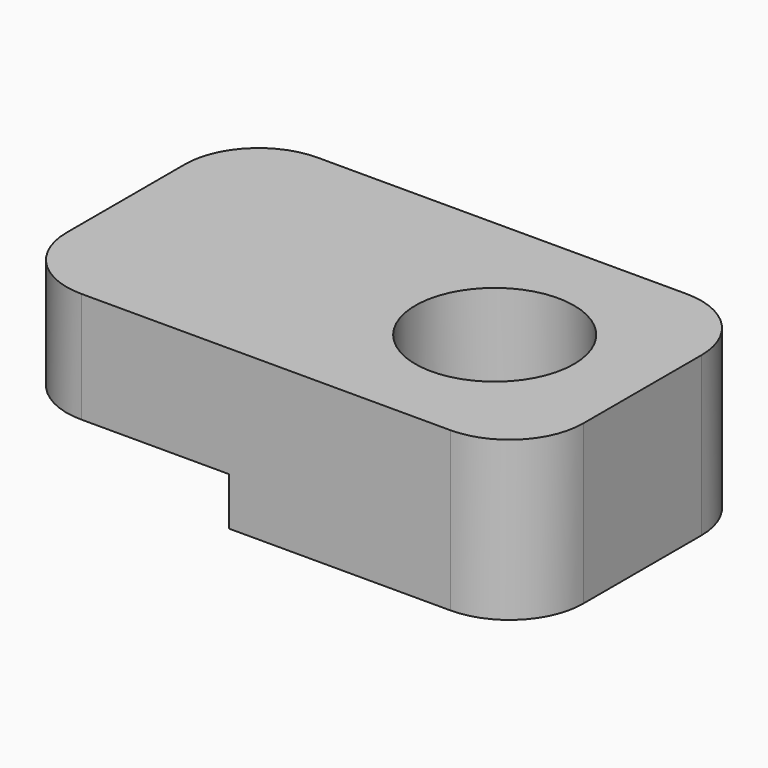
from build123d import *

# Parameters (mm, degrees)
F2_DEPTH = 8
F3_R     = 2.15
F4_DEPTH = 4.3
F5_R     = 2


# Not quite as in the source:
# - a feature names something its author has since deleted; it is built from what else it names


with BuildPart() as f2:
    # F1 (on Front) → F2 (new body)
    with BuildSketch(Plane.XZ):
        Polygon((6, -3), (6, -4.3), (14, -4.3), (14, 0), (0, 0), (0, -3), align=None)
    extrude(amount=F2_DEPTH)

    # F3 (on face) → F4 (cut, through all)
    with BuildSketch(Plane.XY):
        with Locations((10, -4)):
            Circle(F3_R)
    extrude(amount=-F4_DEPTH, mode=Mode.SUBTRACT)

    # F5
    f5_edges = [f2.edges().sort_by_distance(p)[0] for p in [
        (14, -8, -2.15),
        (14, 0, -2.15),
        (0, -8, -1.5),
        (0, 0, -1.5),
    ]]
    fillet(f5_edges, radius=F5_R)


solid = f2.part
